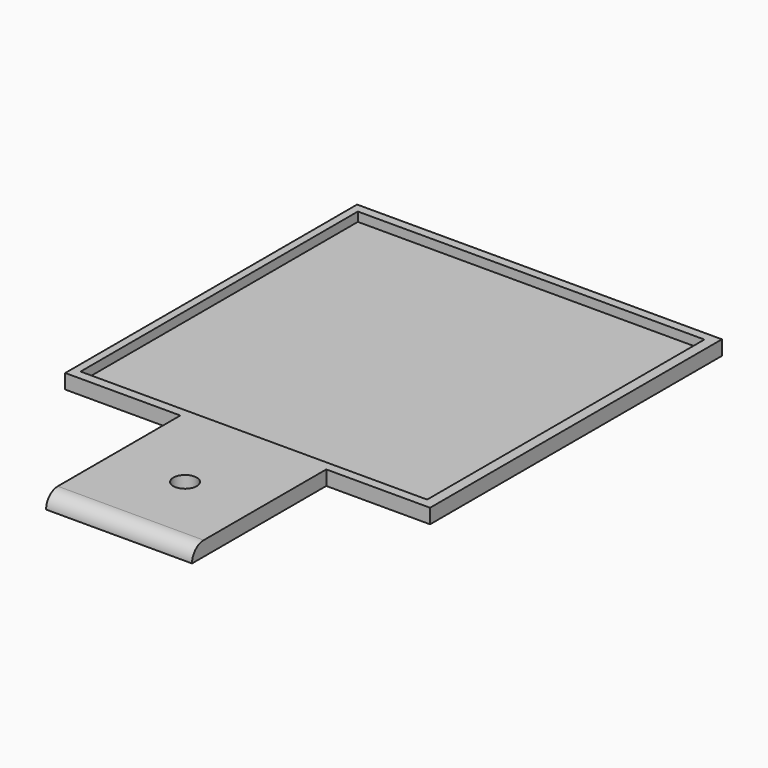
from build123d import *

# Parameters (mm, degrees)
F0_W      = 127
F0_H      = 127
F2_DEPTH  = 5.08
F3_W      = 50.8
F3_H      = 58.42
F4_DEPTH  = 5.08
F5_W      = 50.8
F5_H      = 12.7
F6_DEPTH  = 2.54
F7_R      = 5.07999
F9_W      = 120.65
F9_H      = 120.65
F10_DEPTH = 3.175
F11_R     = 4.064
F12_DEPTH = 25.4


# Not quite as in the source:
# - a fillet or chamfer is up to 0.001 mm smaller than in the source, because OpenCascade refuses the exact size


with BuildPart() as f2:
    # F0 (on Top) → F2 (new body)
    with BuildSketch(Plane.XY):
        with Locations((-1.9660266274, -3.4333672374)):
            Rectangle(F0_W, F0_H)
    extrude(amount=-F2_DEPTH)

    # F3 (on face) → F4 (join)
    with BuildSketch(Plane.XY):
        with Locations((0, -96.1433672374)):
            Rectangle(F3_W, F3_H)
    extrude(amount=-F4_DEPTH)

    # F5 (on face) → F6 (cut)
    with BuildSketch(Plane.XZ.offset(125.3533672374)):
        with Locations((0, -11.43)):
            Rectangle(F5_W, F5_H)
    extrude(amount=-F6_DEPTH, mode=Mode.SUBTRACT)

    # F7 (radius 5.08 in the source; OpenCascade refuses exactly that, so slightly less here)
    f7_edges = [f2.edges().sort_by_distance(p)[0] for p in [
        (0, -125.353367, 0),
    ]]
    fillet(f7_edges, radius=F7_R)

    # F9 (on Top) → F10 (cut)
    with BuildSketch(Plane.XY):
        with Locations((-2.4150442332, -3.342743357)):
            Rectangle(F9_W, F9_H)
    extrude(amount=-F10_DEPTH, mode=Mode.SUBTRACT)

    # F11 (on face) → F12 (cut)
    with BuildSketch(Plane.XY):
        with Locations((0, -96.6428003655)):
            Circle(F11_R)
    extrude(amount=-F12_DEPTH, mode=Mode.SUBTRACT)


solid = f2.part
